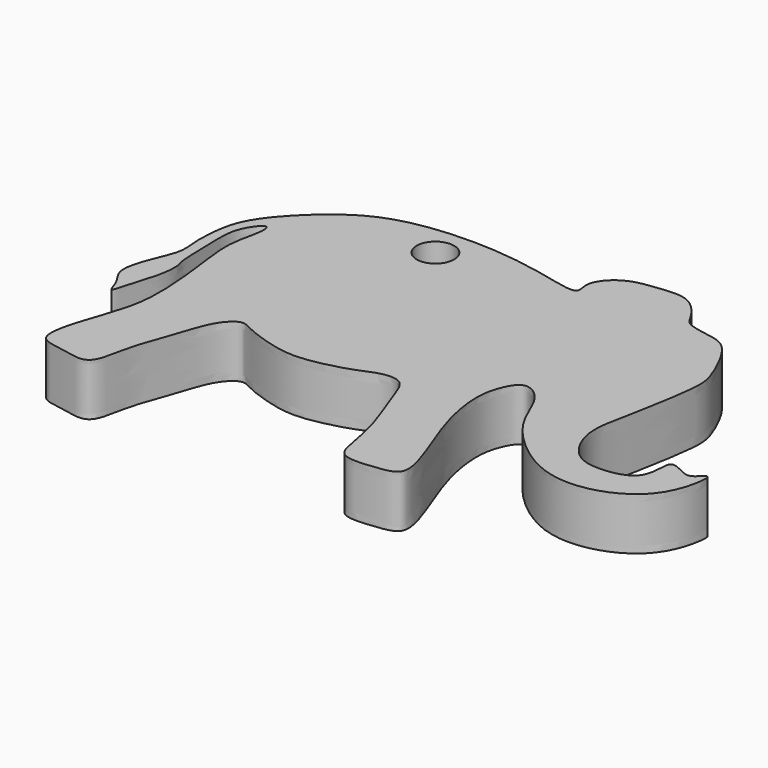
from build123d import *

# Parameters (mm, degrees)
F1_DEPTH = 7
F2_R     = 2.5
F3_DEPTH = 7


with BuildPart() as f1:
    # F0 (on Top) → F1 (new body)
    with BuildSketch(Plane.XY):
        with BuildLine():
            add(Edge.make_bspline(
                [(-38.0405355122, 58.5821075321), (-37.7616920854, 58.8752084321), (-38.4509115224, 60.4144252747), (-36.8912670944, 62.8201922706), (-34.4761482171, 64.0552695288), (-31.741594429, 64.3088112244), (-27.571912684, 64.9103563277), (-24.9592201882, 61.4657628389), (-24.2672174495, 59.7087089783), (-20.270836338, 59.3405969518), (-17.7464919756, 58.2664820468), (-14.9171190454, 52.4096616094), (-14.5229383183, 49.4849582762), (-15.6601088656, 42.8119871017), (-16.4447314113, 38.7626901838), (-17.4306130592, 34.0966946187), (-14.9335226902, 29.1581350963), (-11.036347704, 28.2943890116), (-6.0487945061, 29.3445967564), (-6.1629209222, 33.1615890467), (-5.8426215251, 34.4084166137), (-4.060497983, 33.6421390741), (-2.5204940546, 32.7384503133), (-0.9835052076, 34.8124805933), (-0.8660138479, 33.1705812853), (-1.5192171105, 30.0620356353), (-3.5723199048, 26.7574077509), (-8.1387287813, 24.1006259486), (-15.0993822558, 23.7372030935), (-21.5077719011, 28.5259820845), (-24.376719469, 32.5024508324), (-25.547771341, 36.1152164253), (-27.4169634045, 38.2670221148), (-29.3971839382, 38.6883130727), (-30.7408826881, 36.1727866879), (-31.2951045598, 33.3325303081), (-30.6767268364, 28.6112711634), (-29.0880954099, 23.9986627663), (-27.1266194855, 19.0186140719), (-26.568111716, 16.8817989125), (-26.4774919485, 14.5531424842), (-30.1477398372, 14.1004079283), (-34.2691133605, 13.81975754), (-34.8677649079, 17.3277652031), (-35.8428960167, 22.3235449396), (-38.0725659654, 27.4271356015), (-39.167477751, 31.4476820563), (-42.5748720075, 31.2336825987), (-45.1711193813, 29.8221867938), (-50.8514114479, 28.4276176892), (-54.5233723297, 28.7830868948), (-59.0584026452, 30.2720912872), (-60.9155041476, 31.5925547621), (-63.3541031504, 29.1967940598), (-64.6383866205, 24.322438015), (-66.7606881673, 19.360751826), (-67.3042428271, 13.3420066341), (-71.7158030203, 14.7713797864), (-75.8910666993, 14.9422453013), (-73.9106670496, 21.7940304139), (-71.9694308181, 26.9356793641), (-71.7154077912, 31.9365278137), (-72.3079295729, 38.4192908061), (-73.3304914505, 44.1828607521), (-71.9189568788, 48.4112418783), (-72.4151380297, 50.2824819638), (-74.8686229486, 47.1020249155), (-74.5121986813, 42.9079632641), (-74.5794034955, 38.1004260125), (-73.9785135268, 36.9003015701), (-74.3028735264, 33.7703226695), (-75.3942033439, 31.0657420612), (-76.1293282871, 27.4334387077), (-76.6943195641, 30.3310636229), (-78.6465410892, 32.1249128685), (-77.1724372664, 36.5973140417), (-75.701291774, 39.7127328137), (-76.1770804652, 42.2258292262), (-75.9695046827, 46.5484991401), (-74.8083194931, 49.9948395747), (-70.9728784915, 54.4588701711), (-65.2909207775, 58.9378131806), (-57.8702287571, 60.4837165649), (-50.125383586, 60.5249250526), (-43.3008531913, 59.4158741189), (-38.5069392905, 58.0918561794), (-38.0405355122, 58.5821075321)],
                knots=[0, 0, 0, 0, 0.0079250263, 0.0180756918, 0.0280745586, 0.0383760619, 0.0506316475, 0.0627986403, 0.0709855916, 0.0826585956, 0.0930399111, 0.1081881335, 0.1192950252, 0.1350025479, 0.1479243776, 0.1611538592, 0.174895702, 0.1869669369, 0.1998760516, 0.2110685852, 0.2169307535, 0.2247939205, 0.2328150352, 0.2408713093, 0.2465430974, 0.2577356309, 0.2698241371, 0.2836863731, 0.2996461417, 0.3168271214, 0.3305028043, 0.342422394, 0.3526077963, 0.3603360641, 0.3699749493, 0.3806333359, 0.3938890302, 0.4079437517, 0.4221186114, 0.4314094086, 0.4395117612, 0.4508015917, 0.4626521849, 0.4730671058, 0.4872301942, 0.5021628368, 0.5138814987, 0.5239526556, 0.5348727374, 0.5495348545, 0.5617986993, 0.5751434015, 0.5836517944, 0.5938372003, 0.6077798557, 0.622746205, 0.6361987108, 0.648004278, 0.6590031141, 0.6738305162, 0.688872552, 0.7024907543, 0.7182584033, 0.7334554265, 0.7463776798, 0.7524170519, 0.7627767195, 0.7762202774, 0.7894339564, 0.7965020734, 0.8069266397, 0.8185320821, 0.8279273744, 0.8358727667, 0.8458706014, 0.8587388044, 0.870203602, 0.8798952724, 0.8925416242, 0.9042911544, 0.9190564661, 0.9356398463, 0.9525024072, 0.9696230535, 0.9867443094, 1, 1, 1, 1], degree=3))
        make_face()
    extrude(amount=-F1_DEPTH)

    # F2 (on face) → F3 (cut)
    with BuildSketch(Plane.XY):
        with Locations((-54.9432069991, 56.0719799719)):
            Circle(F2_R)
    extrude(amount=-F3_DEPTH, mode=Mode.SUBTRACT)


solid = f1.part
